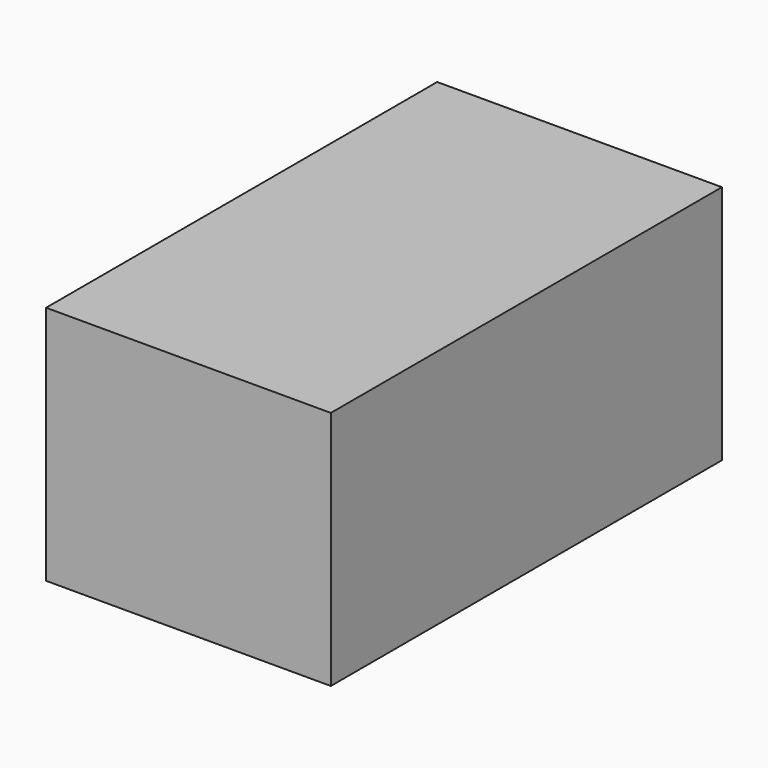
from build123d import *

# Parameters (mm, degrees)
F1_DEPTH = 50.8


# Not quite as in the source:
# - the program builds the solid bodies; features that only make, move or delete a surface that nothing else refers to are left out


with BuildPart() as f1:
    # F0 (on Top) → F1 (new body)
    with BuildSketch(Plane.XY):
        Polygon((-37.3787656426, 57.8591674566), (-97.5454971194, 57.8591674566), (-97.5454971194, -45.4345047474), (-37.3787656426, -45.4345047474), (-37.3787656426, 41.2358790636), align=None)
    extrude(amount=F1_DEPTH)


solid = f1.part
